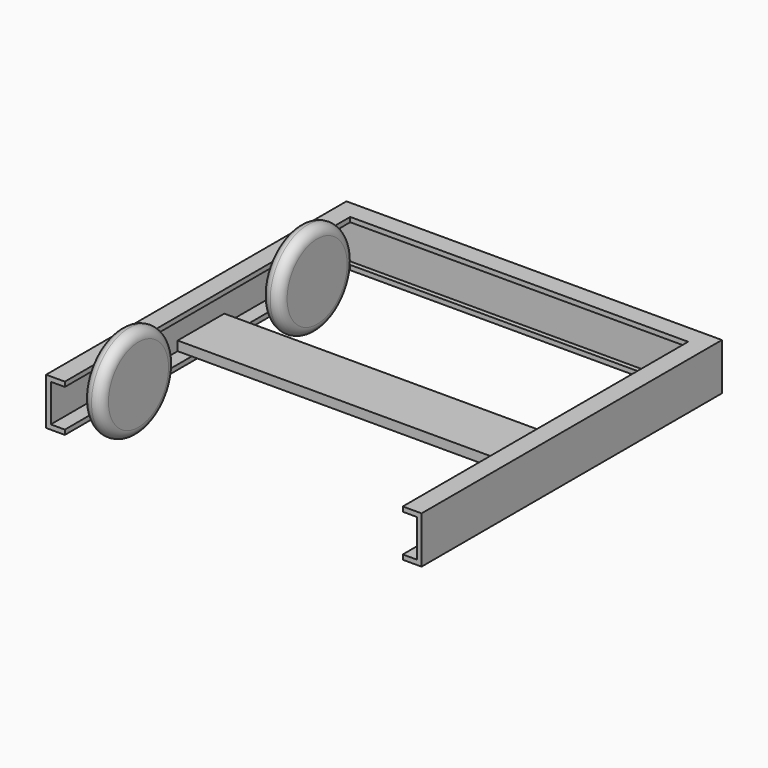
from build123d import *

# Parameters (mm, degrees)
F1_DEPTH  = 12.7
F3_R      = 12.7
F4_DEPTH  = 5.08
F5_R      = 2.53999
F5_2_R    = 2.53999
F8_DEPTH  = 10.16
F9_W      = 99.06
F9_H      = 15.766306633
F10_DEPTH = 2.54


# Not quite as in the source:
# - a fillet or chamfer is up to 0.001 mm smaller than in the source, because OpenCascade refuses the exact size


with BuildPart() as f1:
    # F0 (on Top) → F1 (new body)
    with BuildSketch(Plane.XY):
        Polygon((50.8, -50.8), (50.8, 50.8), (-50.8, 50.8), (-50.8, -50.8), (-45.72, -50.8), (-45.72, -45.72), (-45.72, 45.72), (45.72, 45.72), (45.72, -45.72), (45.72, -50.8), align=None)
    extrude(amount=F1_DEPTH)

    # F7 (on offset) → F8 (cut)
    with BuildSketch(Plane.XY.offset(1.27)):
        Polygon((49.53, 46.99), (-49.53, 46.99), (-49.53, -46.99), (-49.53, -61.8615858257), (49.53, -61.8615858257), (49.53, -46.99), align=None)
    extrude(amount=F8_DEPTH, mode=Mode.SUBTRACT)

    # F9 (on offset) → F10 (join)
    with BuildSketch(Plane.XY.offset(1.27)):
        Rectangle(F9_W, F9_H)
    extrude(amount=F10_DEPTH)


with BuildPart() as f4:
    # F3 (on offset) → F4 (new body)
    with BuildSketch(Plane.YZ.offset(-45.72)):
        with Locations((-32.2580002248, 6.0960003175)):
            Circle(F3_R)
    extrude(amount=F4_DEPTH)

    # F5 (radius 2.54 in the source; OpenCascade refuses exactly that, so slightly less here)
    f5_edges = [f4.edges().sort_by_distance(p)[0] for p in [
        (-40.64, -44.958, 6.096),
        (-45.72, -44.958, 6.096),
    ]]
    fillet(f5_edges, radius=F5_R)


with BuildPart() as f4b:
    # F3 (on offset) → F4, piece 2 (new body)
    with BuildSketch(Plane.YZ.offset(-45.72)):
        with Locations((28.1793344766, 6.0960003175)):
            Circle(F3_R)
    extrude(amount=F4_DEPTH)

    # F5#2 (radius 2.54 in the source; OpenCascade refuses exactly that, so slightly less here)
    f5_2_edges = [f4b.edges().sort_by_distance(p)[0] for p in [
        (-45.72, 15.479334, 6.096),
        (-40.64, 15.479334, 6.096),
    ]]
    fillet(f5_2_edges, radius=F5_2_R)


solid = Compound([f1.part, f4.part, f4b.part])
